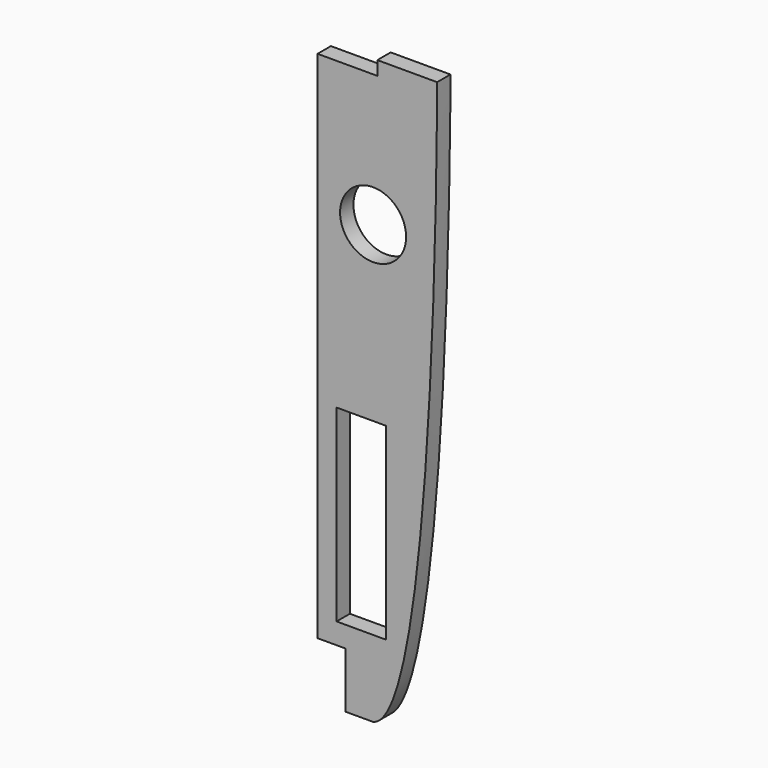
from build123d import *

# Parameters (mm, degrees)
F0_W     = 17.790004611
F0_H     = 67.7184760571
F0_R     = 11.8720680475
F1_DEPTH = 6


# Not quite as in the source:
# - a feature names something its author has since deleted; it is built from what else it names


with BuildPart() as f1:
    # F0 (on Front) → F1 (new body)
    with BuildSketch(Plane.XZ):
        with BuildLine():
            add(Edge.make_bspline(
                [(155.761959786, -128.1328057871), (178.7677402867, -122.1328057871), (178.7677402867, 81.1552154075), (178.761959786, 81.8671942129)],
                knots=[0, 0, 0, 0, 211.255769152, 211.255769152, 211.255769152, 211.255769152], degree=3))
            Line((178.761959786, 81.8671942129), (157.261959786, 81.8671942129))
            Line((157.261959786, 81.8671942129), (157.261959786, 76.8671942129))
            Line((157.261959786, 76.8671942129), (135.761959786, 76.8671942129))
            Line((135.761959786, 76.8671942129), (135.761959786, -108.1328057871))
            Line((135.761959786, -108.1328057871), (145.761959786, -108.1328057871))
            Line((145.761959786, -108.1328057871), (145.761959786, -128.1328057871))
            Line((145.761959786, -128.1328057871), (155.761959786, -128.1328057871))
        make_face()
        with Locations((151.5024825931, -66.7420731425)):
            Rectangle(F0_W, F0_H, mode=Mode.SUBTRACT)
        with Locations((155.7367742062, 29.270966208)):
            Circle(F0_R, mode=Mode.SUBTRACT)
    extrude(amount=F1_DEPTH)


solid = f1.part
